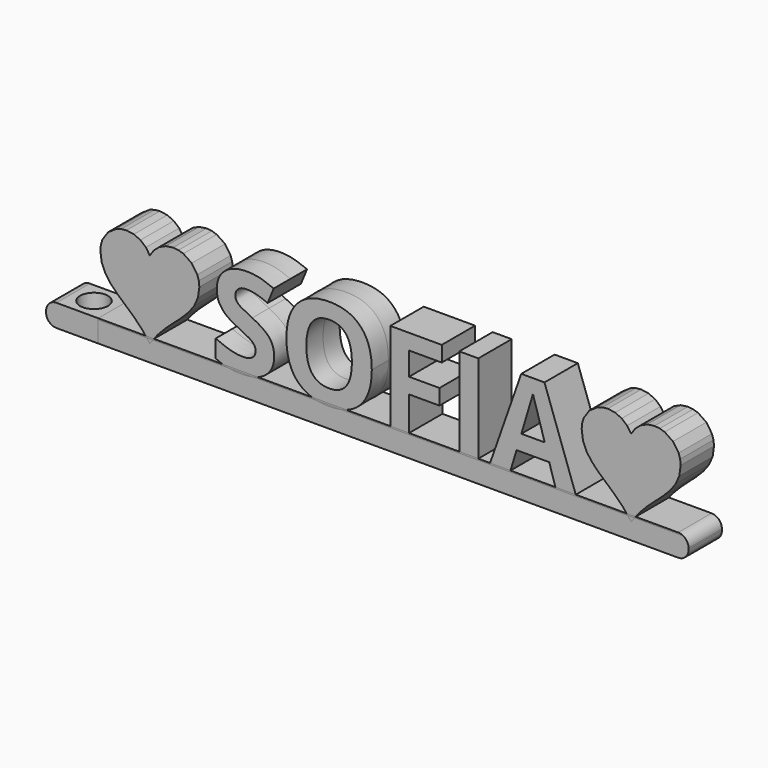
from build123d import *

# Parameters (mm, degrees)
F0_TEXT_SIZE = 18.0798471189
F1_DEPTH     = 3
F2_W         = 85
F2_H         = 6
F3_DEPTH     = 0.2
F4_DEPTH     = 3
F5_W         = 6
F5_H         = 3.2
F6_DEPTH     = 7.5
F7_R         = 1.5
F8_R         = 2
F9_DEPTH     = 4
F10_T1_DEPTH = 13.5


# Not quite as in the source:
# - a fillet or chamfer that OpenCascade refuses, or shapes differently, is made with other operations: its cross-section is extruded or revolved along the edge and cut away or added
# - Text() gives the source's letters only with a copy of the font that has no kerning and outlines rounded to 1/6400 em; it was checked with that copy


with BuildPart() as f1:
    # F0 (on Front) → F1 (new body, symmetric)
    with BuildSketch(Plane.XZ):
        Polygon((54.0351063837, 12.4433699982), (52.9740863837, 12.5970599982), (52.2154763837, 12.5204799982), (51.5086763837, 12.3008699982), (50.3113363837, 11.4933499982), (49.5037163837, 10.2961199982), (49.2840663837, 9.5893599982), (49.2074763837, 8.8307599982), (49.3959963837, 7.3860999982), (49.9167363837, 6.1597099982), (50.7024863837, 5.0814099982), (51.6860163837, 4.0810299982), (53.9828663837, 2.0250499982), (55.1674563837, 0.8247399982), (56.2904463837, -0.5860800018), (56.3347263837, -0.6500000018), (56.3777563837, -0.5851400018), (57.4556663837, 0.8234499982), (58.6189663837, 2.0333299982), (60.9226363837, 4.1212499982), (61.9234263837, 5.1327499982), (62.7284263837, 6.2116199982), (63.2648163837, 7.4226699982), (63.4597963837, 8.8307599982), (63.3832163837, 9.5893599982), (63.1636063837, 10.2961199982), (62.3560863837, 11.4933499982), (61.1588563837, 12.3008699982), (60.4520863837, 12.5204799982), (59.6934963837, 12.5970599982), (58.6324763837, 12.4433699982), (57.6914063837, 12.0123599982), (56.9114563837, 11.3491699982), (56.3337863837, 10.4989199982), (55.7561263837, 11.3491699982), (54.9761763837, 12.0123599982), align=None)
        Polygon((-15.2581707838, 12.5082299799), (-16.3191907838, 12.6619199799), (-17.0778007838, 12.5853399799), (-17.7846007838, 12.3657299799), (-18.9819407838, 11.5582099799), (-19.7895607838, 10.3609799799), (-20.0092107838, 9.6542199799), (-20.0858007838, 8.8956199799), (-19.8972807838, 7.4509599799), (-19.3765407838, 6.2245699799), (-18.5907907838, 5.1462699799), (-17.6072607838, 4.1458899799), (-15.3104107838, 2.0899099799), (-14.1258207838, 0.8895999799), (-13.0028307838, -0.5212200201), (-12.9585507838, -0.5851400201), (-12.9155207838, -0.5202800201), (-11.8376107838, 0.8883099799), (-10.6743107838, 2.0981899799), (-8.3706407838, 4.1861099799), (-7.3698507838, 5.1976099799), (-6.5648507838, 6.2764799799), (-6.0284607838, 7.4875299799), (-5.8334807838, 8.8956199799), (-5.9100607838, 9.6542199799), (-6.1296707838, 10.3609799799), (-6.9371907838, 11.5582099799), (-8.1344207838, 12.3657299799), (-8.8411907838, 12.5853399799), (-9.5997807838, 12.6619199799), (-10.6608007838, 12.5082299799), (-11.6018707838, 12.0772199799), (-12.3818207838, 11.4140299799), (-12.9594907838, 10.5637799799), (-13.5371507838, 11.4140299799), (-14.3171007838, 12.0772199799), align=None)
        with Locations((-4.3061941756, 0)):
            Text('SOFIA', F0_TEXT_SIZE, font='Open Sans', font_style=FontStyle.BOLD, text_align=(TextAlign.LEFT, TextAlign.BOTTOM))
    extrude(amount=F1_DEPTH, both=True)



with BuildPart() as f3:
    # F2 (on Top) → F3 (new body)
    with BuildSketch(Plane.XY):
        with Locations((22.1, 0)):
            Rectangle(F2_W, F2_H)
    extrude(amount=F3_DEPTH)


with BuildPart() as f4:
    # F4 (new): a face of the model
    f4_faces = [f3.part.faces().sort_by_distance(p)[0] for p in [
        (22.1, 0, 0),
    ]]
    extrude(f4_faces, amount=F4_DEPTH)


with BuildPart() as f1_1:
    add(f1.part)

    add(f3.part)  # F6 merges F3

    add(f4.part)  # F6 merges F4
    # F5 (on face) → F6 (join)
    with BuildSketch(Plane(origin=(-20.4, 0, 0), x_dir=(0, -1, 0), z_dir=(-1, 0, 0))):
        with Locations((0, -1.4)):
            Rectangle(F5_W, F5_H)
    extrude(amount=F6_DEPTH)

    # F7
    f7_edges = [f1_1.edges().sort_by_distance(p)[0] for p in [
        (-27.9, 0, -3),
        (-27.9, 0, 0.2),
        (64.6, 0, -3),
    ]]
    fillet(f7_edges, radius=F7_R)

    # F8 (on face) → F9 (cut)
    with BuildSketch(Plane.XY.offset(0.2)):
        with Locations((-23.4, 0)):
            Circle(F8_R)
    extrude(amount=-F9_DEPTH, mode=Mode.SUBTRACT)

    # F10: fillet of radius 1.5 on 1 edges, made by hand

    # F10_s2 → F10_t1 (cut)
    with BuildSketch(Plane.XZ.offset(-6.75)):
        with BuildLine():
            ThreePointArc((64.6, -1.3), (64.1606601718, -0.2393398282), (63.1, 0.2))
            Line((63.1, 0.2), (64.6, 0.2))
            Line((64.6, 0.2), (64.6, -1.3))
        make_face()
    extrude(amount=F10_T1_DEPTH, mode=Mode.SUBTRACT)


solid = f1_1.part
